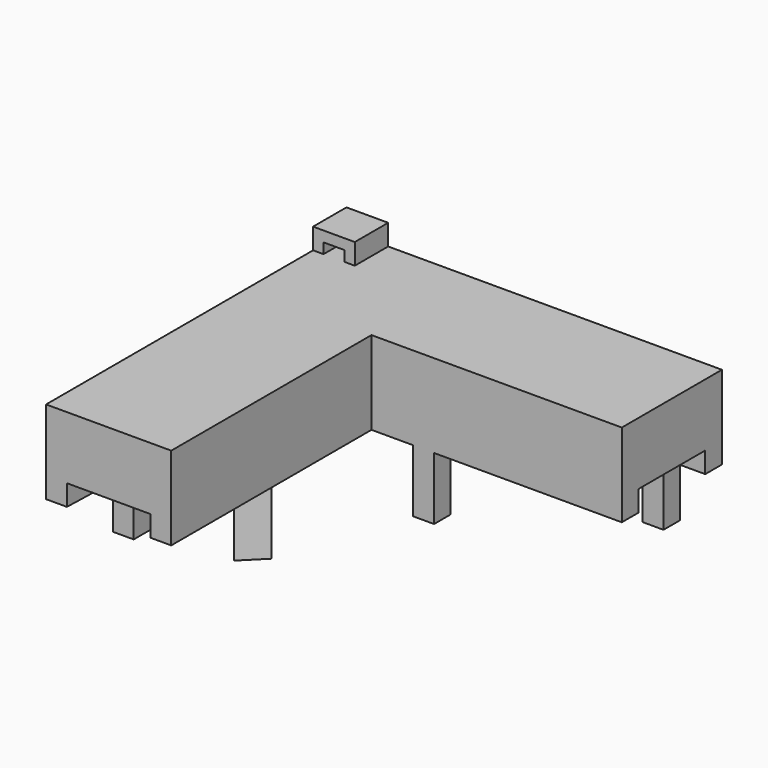
from build123d import *

# Parameters (mm, degrees)
F0_W      = 60
F0_H      = 30
F0_W_2    = 30
F0_H_2    = 60
F1_DEPTH  = 20
F3_DEPTH  = 5
F4_W      = 5
F4_H      = 5
F5_DEPTH  = 15
F6_W      = 5
F6_H      = 5
F7_DEPTH  = 15
F8_DEPTH  = 15
F9_W      = 5
F9_H      = 5
F10_DEPTH = 15
F11_W     = 10
F11_H     = 10
F12_DEPTH = 5
F13_W     = 5
F13_H     = 2.5
F14_DEPTH = 40
F15_DEPTH = 15


# Not quite as in the source:
# - a feature names something its author has since deleted; it is built from what else it names


with BuildPart() as f1:
    # F0 (on Top) → F1 (new body)
    with BuildSketch(Plane.XY):
        with Locations((15, 30)):
            Rectangle(F0_W, F0_H)
        with Locations((-30, 30)):
            Rectangle(F0_W_2, F0_H)
        with Locations((-30, -15)):
            Rectangle(F0_W_2, F0_H_2)
    extrude(amount=F1_DEPTH)

    # F2 (on face) → F3 (cut)
    with BuildSketch(Plane(origin=(0, 0, 0), x_dir=(1, 0, 0), z_dir=(0, 0, -1))):
        Polygon((-13.218164444, -40), (45, -40), (45, -20), (-15, -20), (-20, -20), (-20, -15), (-20, 3.0019930564), (-20, 45), (-40, 45), (-37.5, -40), align=None)
    extrude(amount=-F3_DEPTH, mode=Mode.SUBTRACT)

    # F4 (on face) → F5 (join)
    with BuildSketch(Plane(origin=(0, 0, 0), x_dir=(1, 0, 0), z_dir=(0, 0, -1))):
        with Locations((32.5, -42.5)):
            Rectangle(F4_W, F4_H)
    extrude(amount=F5_DEPTH)

    # F6 (on face) → F7 (join)
    with BuildSketch(Plane(origin=(0, 0, 0), x_dir=(1, 0, 0), z_dir=(0, 0, -1))):
        with Locations((-2.5, -17.5)):
            Rectangle(F6_W, F6_H)
    extrude(amount=F7_DEPTH)

    # F6 (on face) → F8 (join)
    with BuildSketch(Plane(origin=(0, 0, 0), x_dir=(1, 0, 0), z_dir=(0, 0, -1))):
        Polygon((-20, 20), (-20, 15), (-15, 15), align=None)
    extrude(amount=F8_DEPTH)

    # F9 (on face) → F10 (join)
    with BuildSketch(Plane(origin=(0, 0, 0), x_dir=(1, 0, 0), z_dir=(0, 0, -1))):
        with Locations((-42.5, 22.5)):
            Rectangle(F9_W, F9_H)
    extrude(amount=F10_DEPTH)

    # F11 (on face) → F12 (join)
    with BuildSketch(Plane.XY.offset(20)):
        with Locations((-40, 40)):
            Rectangle(F11_W, F11_H)
    extrude(amount=F12_DEPTH)

    # F13 (on face) → F14 (cut)
    with BuildSketch(Plane.XZ.offset(-35)):
        with Locations((-40, 21.25)):
            Rectangle(F13_W, F13_H)
    extrude(amount=-F14_DEPTH, mode=Mode.SUBTRACT)

    # F4 (on face) → F15 (join)
    with BuildSketch(Plane(origin=(0, 0, 0), x_dir=(1, 0, 0), z_dir=(0, 0, -1))):
        with Locations((-42.5, -42.5)):
            Rectangle(F4_W, F4_H)
    extrude(amount=F15_DEPTH)


solid = f1.part
